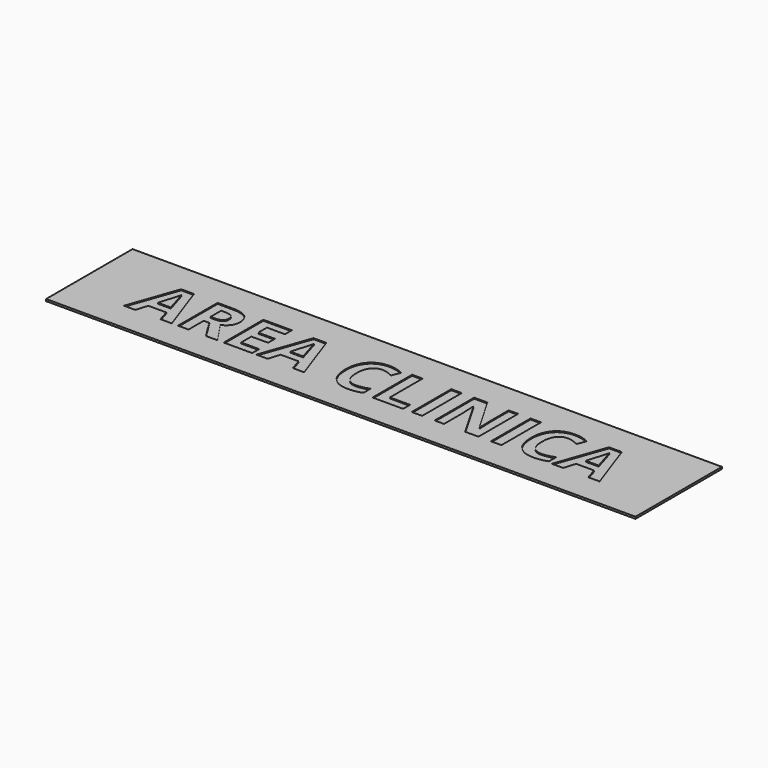
from build123d import *

# Parameters (mm, degrees)
F0_W         = 300
F0_H         = 55
F1_DEPTH     = 1
F2_TEXT_SIZE = 35.2701361955
F3_DEPTH     = 0.5


# Not quite as in the source:
# - Text() gives the source's letters only with a copy of the font that has no kerning and outlines rounded to 1/6400 em; it was checked with that copy


with BuildPart() as f1:
    # F0 (on Top) → F1 (new body)
    with BuildSketch(Plane.XY):
        Rectangle(F0_W, F0_H)
    extrude(amount=F1_DEPTH)

    # F2 (on face) → F3 (cut)
    with BuildSketch(Plane.XY.offset(1)):
        with Locations((-122.2, -12.6944980608)):
            Text('AREA CLINICA', F2_TEXT_SIZE, font='Open Sans', font_style=FontStyle.BOLD, text_align=(TextAlign.LEFT, TextAlign.BOTTOM))
    extrude(amount=-F3_DEPTH, mode=Mode.SUBTRACT)


solid = f1.part
